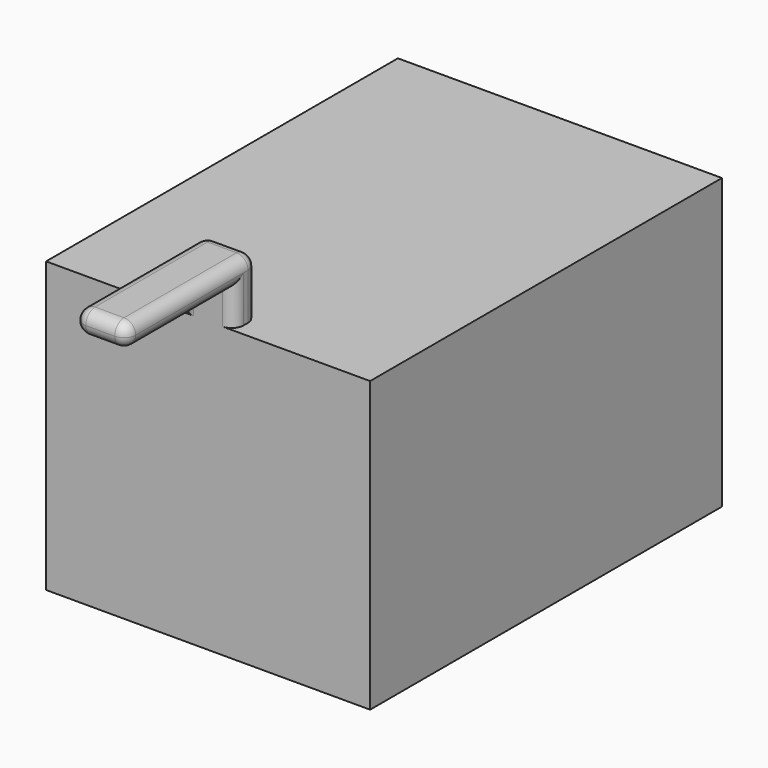
from build123d import *

# Parameters (mm, degrees)
F0_W     = 45
F0_H     = 25
F1_DEPTH = 250
F2_START = 250
F2_DEPTH = 50
F3_START = 280
F3_DEPTH = 20
F4_R     = 9.99999


# Not quite as in the source:
# - a fillet or chamfer is up to 0.001 mm smaller than in the source, because OpenCascade refuses the exact size


with BuildPart() as f1:
    # F0 (on Top) → F1 (new body)
    with BuildSketch(Plane.XY):
        Polygon((0, 380), (0, 0), (117.5, 0), (117.5, 25), (162.5, 25), (162.5, 0), (280, 0), (280, 380), align=None)
        with Locations((140, 12.5)):
            Rectangle(F0_W, F0_H)
    extrude(amount=F1_DEPTH)

    # F0 (on Top) → F2 (join)
    with BuildSketch(Plane.XY.offset(F2_START)):
        with Locations((140, 12.5)):
            Rectangle(F0_W, F0_H)
    extrude(amount=F2_DEPTH)

    # F0 (on Top) → F3 (join)
    with BuildSketch(Plane.XY.offset(F3_START)):
        Polygon((162.5, 0), (117.5, 0), (117.5, -116.4670363069), (140, -116.4670363069), (162.5, -116.4670363069), align=None)
    extrude(amount=F3_DEPTH)

    # F4 (radius 10 in the source; OpenCascade refuses exactly that, so slightly less here)
    f4_edges = [f1.edges().sort_by_distance(p)[0] for p in [
        (140, 25, 300),
        (117.5, -45.733518, 300),
        (162.5, -45.733518, 300),
        (162.5, 25, 275),
        (117.5, 25, 275),
        (162.5, -58.233518, 280),
        (117.5, -58.233518, 280),
        (162.5, 0, 265),
        (117.5, 0, 265),
        (117.5, -116.467036, 290),
        (140, -116.467036, 300),
        (162.5, -116.467036, 290),
        (140, -116.467036, 280),
    ]]
    fillet(f4_edges, radius=F4_R)


solid = f1.part
